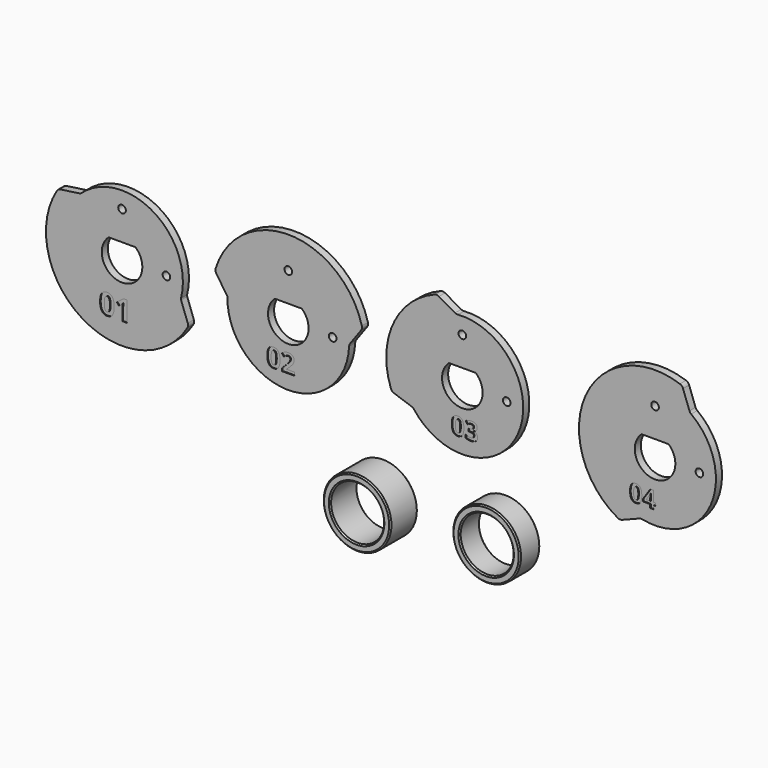
from build123d import *

# Parameters (mm, degrees)
F0_R           = 1.5
F1_DEPTH       = 1.5
F2_TEXT_SIZE   = 11.1464514501
F2_TEXT_SIZE_2 = 10.0362619075
F2_TEXT_SIZE_3 = 9.554099395
F2_TEXT_SIZE_4 = 9.278808203
F3_DEPTH       = 0.3
F4_R           = 13.35
F4_R_2         = 10.45
F5_DEPTH       = 13.5
F6_SIZE        = 0.5
F7_R           = 13.35
F7_R_2         = 10.45
F8_DEPTH       = 5
F9_SIZE        = 0.5


# Not quite as in the source:
# - ends of sketch curves that miss each other by under 0.0002 mm in the source are joined
# - Text() gives the source's letters only with a copy of the font that has no kerning and outlines rounded to 1/6400 em; it was checked with that copy


with BuildPart() as f1:
    # F0 (on Front) → F1 (new body, symmetric)
    with BuildSketch(Plane.XZ):
        with BuildLine():
            ThreePointArc((-78.8256638229, -5.907402045), (-89.8652537727, 20.6548341237), (-118.4617985243, 17.5463674902))
            Line((-118.4617985243, 17.5463674902), (-126.346764, 16.435201))
            ThreePointArc((-126.346764, 16.435201), (-127.170691487, 16.1231098667), (-127.7805633782, 15.487253228))
            ThreePointArc((-127.7805633782, 15.487253228), (-117.528802495, -25.7207943016), (-76.3390557428, -15.3957511538))
            ThreePointArc((-76.3390557428, -15.3957511538), (-76.0645710086, -14.5585441806), (-76.1764747122, -13.6846248951))
            Line((-76.1764747122, -13.6846248951), (-78.795995, -6.495916))
            ThreePointArc((-78.795995, -6.495916), (-78.8551626363, -6.203893962), (-78.8256638229, -5.907402045))
        make_face()
        with BuildLine():
            Line((-107.378779, 6), (-96.795774, 6))
            ThreePointArc((-96.795774, 6), (-102.087275625, -8), (-107.378779, 6))
        make_face(mode=Mode.SUBTRACT)
        with Locations((-84.587276, 0)):
            Circle(F0_R, mode=Mode.SUBTRACT)
        with Locations((-102.087276, 17.5)):
            Circle(F0_R, mode=Mode.SUBTRACT)
    extrude(amount=F1_DEPTH, both=True)


with BuildPart() as f1b:
    # F0 (on Front) → F1, piece 2 (new body, symmetric)
    with BuildSketch(Plane.XZ):
        with BuildLine():
            Line((-64.914103, 7.257761), (-60.516615, 0.619276))
            ThreePointArc((-60.516615, 0.619276), (-37.3353758369, -23.9863013462), (-12.5455407329, -1.0022120112))
            ThreePointArc((-12.5455407329, -1.0022120112), (-12.4362000588, -0.4284601328), (-12.1657594849, 0.0892353521))
            Line((-12.1657594849, 0.0892353521), (-7.850056, 6.033965))
            ThreePointArc((-7.850056, 6.033965), (-7.5022072795, 6.8434455388), (-7.5359521417, 7.7238539622))
            ThreePointArc((-7.5359521417, 7.7238539622), (-35.8813740464, 29.9931034182), (-65.1554678394, 8.9595619498))
            ThreePointArc((-65.1554678394, 8.9595619498), (-65.2269269562, 8.0814102474), (-64.914103, 7.257761))
        make_face()
        with BuildLine():
            Line((-41.816109, 6), (-31.233104, 6))
            ThreePointArc((-31.233104, 6), (-36.524605625, -8), (-41.816109, 6))
        make_face(mode=Mode.SUBTRACT)
        with Locations((-19.024606, 0)):
            Circle(F0_R, mode=Mode.SUBTRACT)
        with Locations((-36.524606, 17.5)):
            Circle(F0_R, mode=Mode.SUBTRACT)
    extrude(amount=F1_DEPTH, both=True)


with BuildPart() as f1c:
    # F0 (on Front) → F1, piece 3 (new body, symmetric)
    with BuildSketch(Plane.XZ):
        with BuildLine():
            ThreePointArc((22.8629012644, 27.8071624678), (22.0192466435, 28.0611389006), (21.1483179088, 27.9279462326))
            ThreePointArc((21.1483179088, 27.9279462326), (4.7466635998, 12.3113375455), (3.9355044716, -10.3212661936))
            ThreePointArc((3.9355044716, -10.3212661936), (4.4133980453, -11.061452027), (5.1629841386, -11.5244615969))
            Line((5.1629841386, -11.5244615969), (12.109746, -13.913519))
            ThreePointArc((12.109746, -13.913519), (12.6284173648, -14.1820838873), (13.0473797399, -14.5890454336))
            ThreePointArc((13.0473797399, -14.5890454336), (53.9901030674, -9.8490701537), (30.3853929972, 23.9383780385))
            ThreePointArc((30.3853929972, 23.9383780385), (29.8029515513, 23.9820660356), (29.257969164, 24.1921632901))
            Line((29.257969164, 24.1921632901), (22.8629012644, 27.8071624678))
        make_face()
        with BuildLine():
            Line((26.812628, 6), (37.395633, 6))
            ThreePointArc((37.395633, 6), (32.104129625, -8), (26.812628, 6))
        make_face(mode=Mode.SUBTRACT)
        with Locations((49.60413, 0)):
            Circle(F0_R, mode=Mode.SUBTRACT)
        with Locations((32.10413, 17.5)):
            Circle(F0_R, mode=Mode.SUBTRACT)
    extrude(amount=F1_DEPTH, both=True)


with BuildPart() as f1d:
    # F0 (on Front) → F1, piece 4 (new body, symmetric)
    with BuildSketch(Plane.XZ):
        with BuildLine():
            ThreePointArc((101.9195359991, -23.5652369977), (102.488355494, -23.432605817), (103.0712369264, -23.4699673444))
            ThreePointArc((103.0712369264, -23.4699673444), (129.9732500123, -9.8490702761), (122.3270719424, 19.3191159218))
            ThreePointArc((122.3270719424, 19.3191159218), (121.9125530979, 19.7306021195), (121.634592595, 20.2442992168))
            Line((121.634592595, 20.2442992168), (119.119499, 27.14643))
            ThreePointArc((119.119499, 27.14643), (118.6429234543, 27.8874653165), (117.8941618877, 28.3518076754))
            ThreePointArc((117.8941618877, 28.3518076754), (80.7298105994, 12.3113375447), (93.370811959, -26.1424110728))
            ThreePointArc((93.370811959, -26.1424110728), (94.2149171416, -26.3948867917), (95.0856078663, -26.2601446611))
            Line((95.0856078663, -26.2601446611), (101.9195359991, -23.5652369977))
        make_face()
        with BuildLine():
            Line((102.795775, 6), (113.37878, 6))
            ThreePointArc((113.37878, 6), (108.087276625, -8), (102.795775, 6))
        make_face(mode=Mode.SUBTRACT)
        with Locations((125.587277, 0)):
            Circle(F0_R, mode=Mode.SUBTRACT)
        with Locations((108.087277, 17.5)):
            Circle(F0_R, mode=Mode.SUBTRACT)
    extrude(amount=F1_DEPTH, both=True)


with BuildPart() as f3_tool:
    # F2 (on face) → F3 (new body)
    with BuildSketch(Plane.XZ.offset(1.5)):
        with Locations((-111.1393421888, -21.3850513101)):
            Text('01', F2_TEXT_SIZE, font='Open Sans', font_style=FontStyle.BOLD, text_align=(TextAlign.LEFT, TextAlign.BOTTOM))
        with Locations((-45.1696813107, -18.2617194951)):
            Text('02', F2_TEXT_SIZE_2, font='Open Sans', font_style=FontStyle.BOLD, text_align=(TextAlign.LEFT, TextAlign.BOTTOM))
        with Locations((27.5971442461, -18.1958209723)):
            Text('03', F2_TEXT_SIZE_3, font='Open Sans', font_style=FontStyle.BOLD, text_align=(TextAlign.LEFT, TextAlign.BOTTOM))
        with Locations((97.9086458683, -18.5865536332)):
            Text('04', F2_TEXT_SIZE_4, font='Open Sans', font_style=FontStyle.BOLD, text_align=(TextAlign.LEFT, TextAlign.BOTTOM))
    extrude(amount=-F3_DEPTH)


with BuildPart() as f1_1:
    add(f1.part)

    # F3: cut by f3_tool
    add(f3_tool.part, mode=Mode.SUBTRACT)


with BuildPart() as f1b_1:
    add(f1b.part)

    # F3: cut by f3_tool
    add(f3_tool.part, mode=Mode.SUBTRACT)


with BuildPart() as f1c_1:
    add(f1c.part)

    # F3: cut by f3_tool
    add(f3_tool.part, mode=Mode.SUBTRACT)


with BuildPart() as f1d_1:
    add(f1d.part)

    # F3: cut by f3_tool
    add(f3_tool.part, mode=Mode.SUBTRACT)


with BuildPart() as f5:
    # F4 (on Front) → F5 (new body)
    with BuildSketch(Plane.XZ):
        with Locations((0, -50)):
            Circle(F4_R)
        with Locations((0, -50)):
            Circle(F4_R_2, mode=Mode.SUBTRACT)
    extrude(amount=F5_DEPTH)

    # F6
    f6_edges = [f5.edges().sort_by_distance(p)[0] for p in [
        (-10.45, -13.5, -50),
        (-13.35, -13.5, -50),
        (-10.45, 0, -50),
        (-13.35, 0, -50),
    ]]
    chamfer(f6_edges, length=F6_SIZE)


with BuildPart() as f8:
    # F7 (on Front) → F8 (new body, symmetric)
    with BuildSketch(Plane.XZ):
        with Locations((44.2896448076, -50)):
            Circle(F7_R)
        with Locations((44.2896448076, -50)):
            Circle(F7_R_2, mode=Mode.SUBTRACT)
    extrude(amount=F8_DEPTH, both=True)

    # F9
    f9_edges = [f8.edges().sort_by_distance(p)[0] for p in [
        (33.839645, -5, -50),
        (30.939645, -5, -50),
        (30.939645, 5, -50),
        (33.839645, 5, -50),
    ]]
    chamfer(f9_edges, length=F9_SIZE)


solid = Compound([f1_1.part, f1b_1.part, f1c_1.part, f1d_1.part, f5.part, f8.part])
